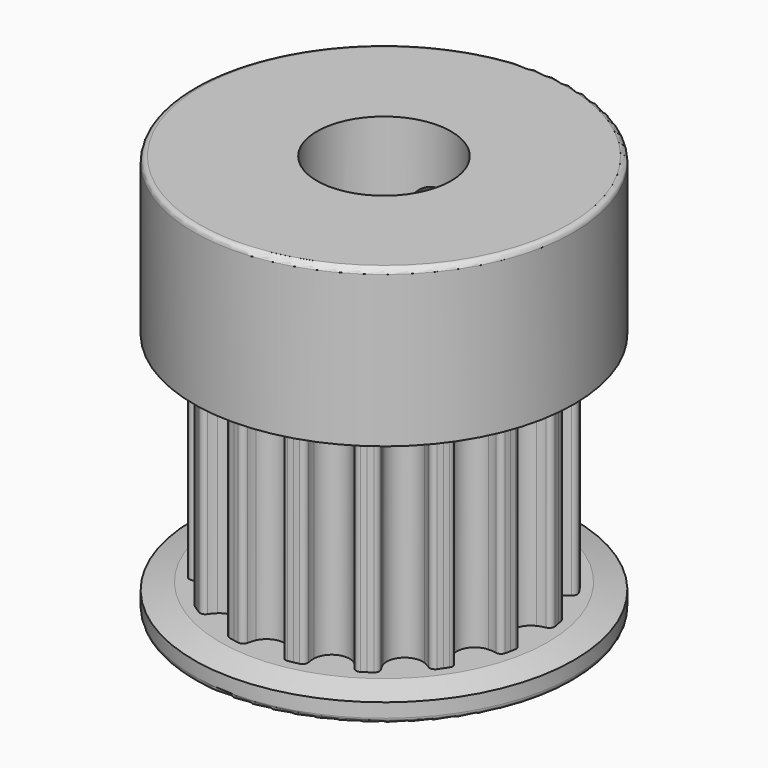
from build123d import *

# Parameters (mm, degrees)
F3_DEPTH    = 5
F4_COUNT    = 16
F5_R        = 9
F6_DEPTH    = 1.25
F7_R        = 9
F8_DEPTH    = 1.25
F9_R        = 9
F10_DEPTH   = 6.5
F11_R       = 3.175
F12_DEPTH   = 19.001
F13_R       = 1.25
F14_DEPTH   = 9.001
F15_R       = 1.25
F16_DEPTH   = 9.0010001
F17_SIZE2   = 0.3349364905
F17_SIZE    = 1.25
F17_2_SIZE2 = 0.3349364905
F17_2_SIZE  = 1.25
F18_R       = 0.25


# Not quite as in the source:
# - a feature names something its author has since deleted; it is built from what else it names


with BuildPart() as f3:
    # F2 (on Top) → F3 (new body, symmetric)
    with BuildSketch(Plane.XY):
        with BuildLine():
            ThreePointArc((0.7729699653, 6.6005393756), (0.459324865, 6.2389106877), (0, 6.1041174189))
            ThreePointArc((0, 6.1041174189), (-0.459324865, 6.2389106877), (-0.7729699653, 6.6005393756))
            ThreePointArc((-0.7729699653, 6.6005393756), (-0.840847916, 6.777273601), (-0.8862292653, 6.9610749495))
            ThreePointArc((-0.8862292653, 6.9610749495), (-0.9880853916, 7.1206605485), (-1.1725886371, 7.1630962207))
            ThreePointArc((-1.1725886371, 7.1630962207), (-1.2945077953, 7.1420698083), (-1.416050864, 7.1189684316))
            Line((-1.416050864, 7.1189684316), (0, 0))
            Line((0, 0), (1.416050864, 7.1189684316))
            ThreePointArc((1.416050864, 7.1189684316), (1.2945077953, 7.1420698083), (1.1725886371, 7.1630962207))
            ThreePointArc((1.1725886371, 7.1630962207), (0.9880853916, 7.1206605485), (0.8862292653, 6.9610749495))
            ThreePointArc((0.8862292653, 6.9610749495), (0.840847916, 6.777273601), (0.7729699653, 6.6005393756))
        make_face()
    extrude(amount=F3_DEPTH, both=True)

    # F4: F3 ×16 about axis
    f4_axis = Axis((0, 0, 0), (0, 0, -1))


with BuildPart() as f3_1:
    add(f3.part)
    for i in range(1, F4_COUNT):
        add(f3.part.rotate(f4_axis, i * 360 / F4_COUNT))

    # F5 (on face) → F6 (join)
    with BuildSketch(Plane(origin=(0, 0, -5), x_dir=(1, 0, 0), z_dir=(0, 0, -1))):
        Circle(F5_R)
    extrude(amount=F6_DEPTH)

    # F7 (on face) → F8 (join)
    with BuildSketch(Plane.XY.offset(5)):
        Circle(F7_R)
    extrude(amount=F8_DEPTH)

    # F9 (on face) → F10 (join)
    with BuildSketch(Plane.XY.offset(6.25)):
        Circle(F9_R)
    extrude(amount=F10_DEPTH)

    # F11 (on face) → F12 (cut, through all)
    with BuildSketch(Plane.XY.offset(12.75)):
        Circle(F11_R)
    extrude(amount=-F12_DEPTH, mode=Mode.SUBTRACT)

    # F13 (on Front) → F14 (cut, through all)
    with BuildSketch(Plane.XZ):
        with Locations((0, 8.875)):
            Circle(F13_R)
    extrude(amount=-F14_DEPTH, mode=Mode.SUBTRACT)

    # F15 (on Right) → F16 (cut, through all)
    with BuildSketch(Plane.YZ):
        with Locations((0, 8.875)):
            Circle(F15_R)
    extrude(amount=-F16_DEPTH, mode=Mode.SUBTRACT)

    # F17
    f17_edges = [f3_1.edges().sort_by_distance(p)[0] for p in [
        (-9, 0, -5),
    ]]
    f17_side = f3_1.faces().sort_by_distance((-8.745442, 0, -5))[0]
    chamfer(f17_edges, length=F17_SIZE, length2=F17_SIZE2, reference=f17_side)

    # F17#2
    f17_2_edges = [f3_1.edges().sort_by_distance(p)[0] for p in [
        (-9, 0, 5),
    ]]
    f17_2_side = f3_1.faces().sort_by_distance((-8.745442, 0, 5))[0]
    chamfer(f17_2_edges, length=F17_2_SIZE, length2=F17_2_SIZE2, reference=f17_2_side)

    # F18
    f18_edges = [f3_1.edges().sort_by_distance(p)[0] for p in [
        (-9, 0, 12.75),
        (-9, 0, -6.25),
    ]]
    fillet(f18_edges, radius=F18_R)


solid = f3_1.part
